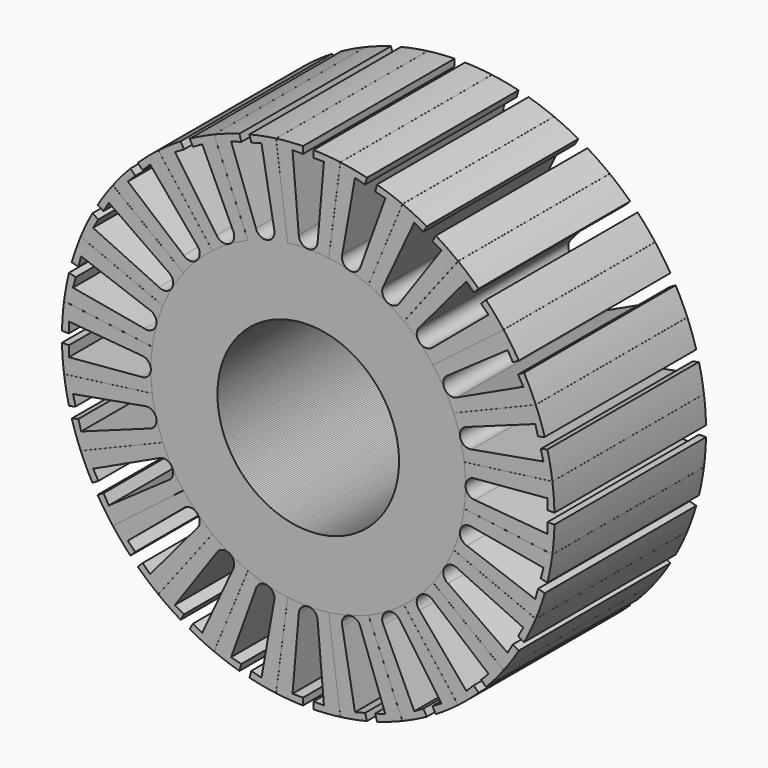
from build123d import *

# Parameters (mm, degrees)
F0_R     = 24
F1_DEPTH = 50
F2_COUNT = 24


with BuildPart() as f1:
    # F0 (on Front) → F1 (new body)
    with BuildSketch(Plane.XZ):
        with BuildLine():
            Line((-8.4783722932, 64.4446832815), (-5.4170277129, 41.1751953336))
            ThreePointArc((-5.4170277129, 41.1751953336), (0, -41.53), (5.4170277129, 41.1751953336))
            Line((5.4170277129, 41.1751953336), (8.4783722932, 64.4446832815))
            ThreePointArc((8.4783722932, 64.4446832815), (4.9341002146, 64.8124575608), (1.375, 64.9854551034))
            Line((1.375, 64.9854551034), (1.375, 63.16))
            Line((1.375, 63.16), (4.15, 63.16))
            Line((4.15, 63.16), (2.49, 44.02))
            ThreePointArc((2.49, 44.02), (0, 41.53), (-2.49, 44.02))
            Line((-2.49, 44.02), (-4.15, 63.16))
            Line((-4.15, 63.16), (-1.375, 63.16))
            Line((-1.375, 63.16), (-1.375, 64.9854551034))
            ThreePointArc((-1.375, 64.9854551034), (-4.9341002146, 64.8124575608), (-8.4783722932, 64.4446832815))
        make_face()
        Circle(F0_R, mode=Mode.SUBTRACT)
    extrude(amount=F1_DEPTH)


with BuildPart() as f2_1:
    # F2: instance of F1
    add(f1.part.rotate(Axis((0, 0, 0), (0, 1, 0)), 1 * 360 / F2_COUNT))


with BuildPart() as f2_2:
    # F2: instance of F1
    add(f1.part.rotate(Axis((0, 0, 0), (0, 1, 0)), 2 * 360 / F2_COUNT))


with BuildPart() as f2_3:
    # F2: instance of F1
    add(f1.part.rotate(Axis((0, 0, 0), (0, 1, 0)), 3 * 360 / F2_COUNT))


with BuildPart() as f2_4:
    # F2: instance of F1
    add(f1.part.rotate(Axis((0, 0, 0), (0, 1, 0)), 4 * 360 / F2_COUNT))


with BuildPart() as f2_5:
    # F2: instance of F1
    add(f1.part.rotate(Axis((0, 0, 0), (0, 1, 0)), 5 * 360 / F2_COUNT))


with BuildPart() as f2_6:
    # F2: instance of F1
    add(f1.part.rotate(Axis((0, 0, 0), (0, 1, 0)), 6 * 360 / F2_COUNT))


with BuildPart() as f2_7:
    # F2: instance of F1
    add(f1.part.rotate(Axis((0, 0, 0), (0, 1, 0)), 7 * 360 / F2_COUNT))


with BuildPart() as f2_8:
    # F2: instance of F1
    add(f1.part.rotate(Axis((0, 0, 0), (0, 1, 0)), 8 * 360 / F2_COUNT))


with BuildPart() as f2_9:
    # F2: instance of F1
    add(f1.part.rotate(Axis((0, 0, 0), (0, 1, 0)), 9 * 360 / F2_COUNT))


with BuildPart() as f2_10:
    # F2: instance of F1
    add(f1.part.rotate(Axis((0, 0, 0), (0, 1, 0)), 10 * 360 / F2_COUNT))


with BuildPart() as f2_11:
    # F2: instance of F1
    add(f1.part.rotate(Axis((0, 0, 0), (0, 1, 0)), 11 * 360 / F2_COUNT))


with BuildPart() as f2_12:
    # F2: instance of F1
    add(f1.part.rotate(Axis((0, 0, 0), (0, 1, 0)), 12 * 360 / F2_COUNT))


with BuildPart() as f2_13:
    # F2: instance of F1
    add(f1.part.rotate(Axis((0, 0, 0), (0, 1, 0)), 13 * 360 / F2_COUNT))


with BuildPart() as f2_14:
    # F2: instance of F1
    add(f1.part.rotate(Axis((0, 0, 0), (0, 1, 0)), 14 * 360 / F2_COUNT))


with BuildPart() as f2_15:
    # F2: instance of F1
    add(f1.part.rotate(Axis((0, 0, 0), (0, 1, 0)), 15 * 360 / F2_COUNT))


with BuildPart() as f2_16:
    # F2: instance of F1
    add(f1.part.rotate(Axis((0, 0, 0), (0, 1, 0)), 16 * 360 / F2_COUNT))


with BuildPart() as f2_17:
    # F2: instance of F1
    add(f1.part.rotate(Axis((0, 0, 0), (0, 1, 0)), 17 * 360 / F2_COUNT))


with BuildPart() as f2_18:
    # F2: instance of F1
    add(f1.part.rotate(Axis((0, 0, 0), (0, 1, 0)), 18 * 360 / F2_COUNT))


with BuildPart() as f2_19:
    # F2: instance of F1
    add(f1.part.rotate(Axis((0, 0, 0), (0, 1, 0)), 19 * 360 / F2_COUNT))


with BuildPart() as f2_20:
    # F2: instance of F1
    add(f1.part.rotate(Axis((0, 0, 0), (0, 1, 0)), 20 * 360 / F2_COUNT))


with BuildPart() as f2_21:
    # F2: instance of F1
    add(f1.part.rotate(Axis((0, 0, 0), (0, 1, 0)), 21 * 360 / F2_COUNT))


with BuildPart() as f2_22:
    # F2: instance of F1
    add(f1.part.rotate(Axis((0, 0, 0), (0, 1, 0)), 22 * 360 / F2_COUNT))


with BuildPart() as f2_23:
    # F2: instance of F1
    add(f1.part.rotate(Axis((0, 0, 0), (0, 1, 0)), 23 * 360 / F2_COUNT))


solid = Compound([f1.part, f2_1.part, f2_2.part, f2_3.part, f2_4.part, f2_5.part, f2_6.part, f2_7.part, f2_8.part, f2_9.part, f2_10.part, f2_11.part, f2_12.part, f2_13.part, f2_14.part, f2_15.part, f2_16.part, f2_17.part, f2_18.part, f2_19.part, f2_20.part, f2_21.part, f2_22.part, f2_23.part])
